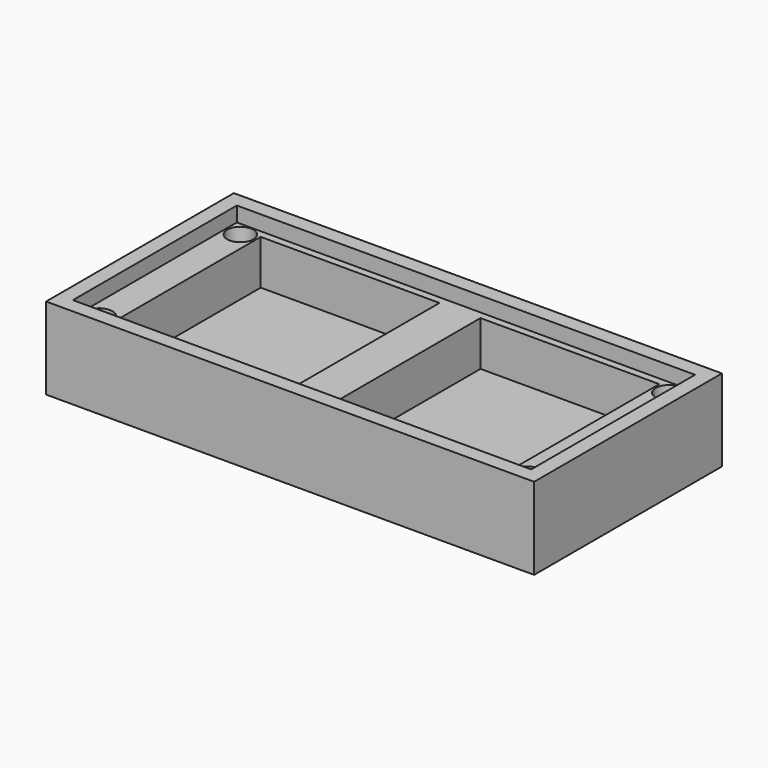
from build123d import *

# Parameters (mm, degrees)
F0_W     = 103.98125
F0_H     = 50.00625
F0_W_2   = 97.63125
F0_H_2   = 43.65625
F0_W_3   = 38.1
F0_H_3   = 40.48125
F1_DEPTH = 4.7625
F2_DEPTH = 14.2875
F3_DEPTH = 17.4625
F4_R     = 2.794
F4_R_2   = 2.032
F5_DEPTH = 3.175
F6_DEPTH = 14.2875


with BuildPart() as f1:
    # F0 (on Top) → F1 (new body)
    with BuildSketch(Plane.XY):
        with Locations((51.990625, 25.003125)):
            Rectangle(F0_W, F0_H)
        with Locations((51.990625, 25.003125)):
            Rectangle(F0_W_2, F0_H_2, mode=Mode.SUBTRACT)
        with Locations((51.990625, 25.003125)):
            Rectangle(F0_W_2, F0_H_2)
        with Locations((28.575, 25.003125)):
            Rectangle(F0_W_3, F0_H_3, mode=Mode.SUBTRACT)
        with Locations((75.40625, 25.003125)):
            Rectangle(F0_W_3, F0_H_3, mode=Mode.SUBTRACT)
        with Locations((28.575, 25.003125)):
            Rectangle(F0_W_3, F0_H_3)
        with Locations((75.40625, 25.003125)):
            Rectangle(F0_W_3, F0_H_3)
    extrude(amount=F1_DEPTH)

    # F0 (on Top) → F2 (join)
    with BuildSketch(Plane.XY):
        with Locations((51.990625, 25.003125)):
            Rectangle(F0_W, F0_H)
        with Locations((51.990625, 25.003125)):
            Rectangle(F0_W_2, F0_H_2, mode=Mode.SUBTRACT)
        with Locations((51.990625, 25.003125)):
            Rectangle(F0_W_2, F0_H_2)
        with Locations((28.575, 25.003125)):
            Rectangle(F0_W_3, F0_H_3, mode=Mode.SUBTRACT)
        with Locations((75.40625, 25.003125)):
            Rectangle(F0_W_3, F0_H_3, mode=Mode.SUBTRACT)
    extrude(amount=F2_DEPTH)

    # F0 (on Top) → F3 (join)
    with BuildSketch(Plane.XY):
        with Locations((51.990625, 25.003125)):
            Rectangle(F0_W, F0_H)
        with Locations((51.990625, 25.003125)):
            Rectangle(F0_W_2, F0_H_2, mode=Mode.SUBTRACT)
    extrude(amount=F3_DEPTH)

    # F4 (on face) → F5 (cut)
    with BuildSketch(Plane.XY.offset(14.2875)):
        with Locations((6.35, 43.799125)):
            Circle(F4_R)
        with Locations((6.35, 43.799125)):
            Circle(F4_R_2, mode=Mode.SUBTRACT)
        with Locations((6.35, 6.207125)):
            Circle(F4_R)
        with Locations((6.35, 6.207125)):
            Circle(F4_R_2, mode=Mode.SUBTRACT)
        with Locations((97.63125, 43.799125)):
            Circle(F4_R)
        with Locations((97.63125, 43.799125)):
            Circle(F4_R_2, mode=Mode.SUBTRACT)
        with Locations((97.63125, 6.207125)):
            Circle(F4_R)
        with Locations((97.63125, 6.207125)):
            Circle(F4_R_2, mode=Mode.SUBTRACT)
    extrude(amount=-F5_DEPTH, mode=Mode.SUBTRACT)

    # F6 (cut, through all): faces of the model
    f6_faces = [f1.faces().sort_by_distance(p)[0] for p in [
        (6.35, 43.799125, 14.2875),
        (97.63125, 43.799125, 14.2875),
        (97.63125, 6.207125, 14.2875),
        (6.35, 6.207125, 14.2875),
    ]]
    extrude(f6_faces, amount=-F6_DEPTH, mode=Mode.SUBTRACT)


solid = f1.part
